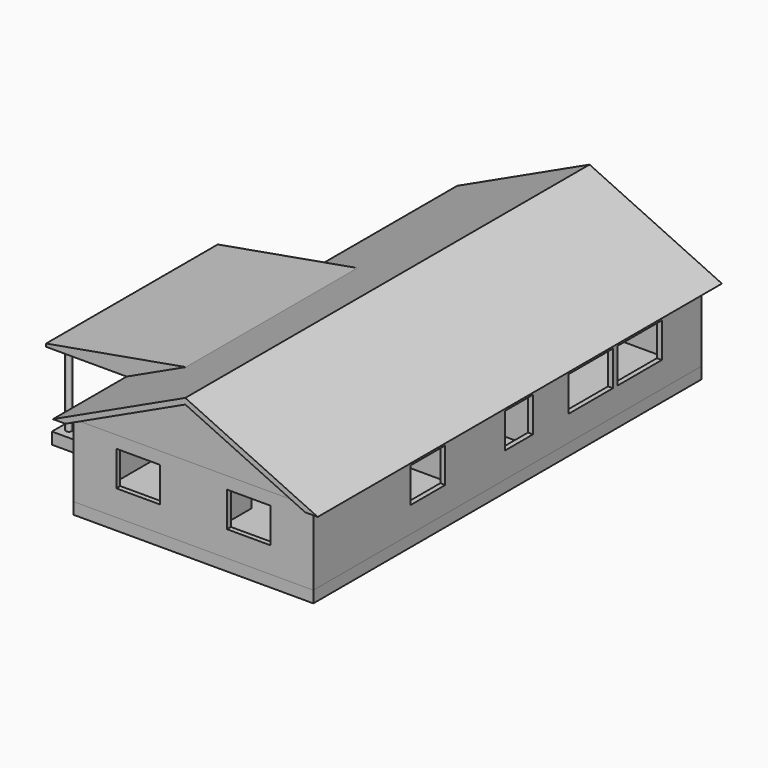
from build123d import *

# Parameters (mm, degrees)
F0_W           = 1130
F0_H           = 1950
F0_W_2         = 1120
F0_H_2         = 1100
F0_W_3         = 3760
F0_H_3         = 1500
F0_W_4         = 1710
F0_H_4         = 2010
F0_W_5         = 850
F0_H_5         = 530
F0_W_6         = 3710
F0_H_6         = 100
F1_DEPTH       = 2500
F3_START       = -400
F2_W           = 170
F2_H           = 850
F2_W_2         = 800
F2_H_2         = 150
F2_W_3         = 880
F2_H_3         = 115
F2_W_4         = 870
F2_W_5         = 850
F2_H_4         = 880
F2_W_6         = 650
F2_H_5         = 100
F2_W_7         = 160
F2_H_6         = 200
F2_W_8         = 100
F3_DEPTH       = 2100
F4_W           = 8250
F4_H           = 16680
F5_DEPTH       = 400
F6_W           = 1100
F6_H           = 650
F6_W_2         = 1350
F6_W_3         = 350
F6_H_2         = 1200
F6_W_4         = 1500
F10_DEPTH      = 170
F7_W           = 1300
F7_H           = 650
F11_DEPTH      = 200
F8_W           = 1200
F8_H           = 1200
F8_W_2         = 1900
F8_W_3         = 1500
F12_DEPTH      = 170
F9_W           = 1500
F9_H           = 1200
F13_DEPTH      = 170
F15_DEPTH      = 16680
F17_DEPTH      = 17030
F17_DEPTH_BACK = 350
F18_W          = 7380
F18_H          = 400
F19_DEPTH      = 3000
F20_W          = 1280
F20_H          = 220
F21_DEPTH      = 400
F22_R          = 100
F23_DEPTH      = 2500
F25_DEPTH      = 7380


# Not quite as in the source:
# - a feature names something its author has since deleted; it is built from what else it names


with BuildPart() as f1:
    # F0 (on Top) → F1 (new body)
    with BuildSketch(Plane.XY):
        Polygon((4125, 0), (-4125, 0), (-4125, -9510), (-3955, -9510), (-245, -9510), (-145, -9510), (3955, -9510), (4125, -9510), align=None)
        with Locations((-3390, -8335)):
            Rectangle(F0_W, F0_H, mode=Mode.SUBTRACT)
        with Locations((-2105, -6980)):
            Rectangle(F0_W_2, F0_H_2, mode=Mode.SUBTRACT)
        Polygon((-3955, -6245), (-3955, -3975), (-195, -3975), (-195, -6245), (-2825, -6245), (-2825, -7245), (-3955, -7245), align=None, mode=Mode.SUBTRACT)
        Polygon((-3955, -3860), (-3955, -1850), (-2105, -1850), (-2105, -3330), (-2105, -3860), (-2955, -3860), align=None, mode=Mode.SUBTRACT)
        with Locations((-2075, -950)):
            Rectangle(F0_W_3, F0_H_3, mode=Mode.SUBTRACT)
        with Locations((-1050, -2855)):
            Rectangle(F0_W_4, F0_H_4, mode=Mode.SUBTRACT)
        Polygon((-45, -6430), (-45, -200), (3955, -200), (3955, -5800), (1905, -5800), (1905, -6490), (3955, -6490), (3955, -9310), (955, -9310), (955, -7290), (805, -7290), (805, -9310), (-2665, -9310), (-2665, -7630), (-1415, -7630), (-1415, -6430), align=None, mode=Mode.SUBTRACT)
        with Locations((-2530, -3595)):
            Rectangle(F0_W_5, F0_H_5)
        Polygon((-145, -9510), (-245, -9510), (-245, -12960), (-245, -13060), (-245, -16510), (-145, -16510), align=None)
        with Locations((-2100, -13010)):
            Rectangle(F0_W_6, F0_H_6)
        Polygon((-3955, -9510), (-4125, -9510), (-4125, -16680), (4125, -16680), (4125, -9510), (3955, -9510), (3955, -16510), (-145, -16510), (-245, -16510), (-3955, -16510), (-3955, -13060), (-3955, -12960), align=None)
    extrude(amount=F1_DEPTH)

    # F2 (on face) → F3 (cut)
    with BuildSketch(Plane.XY.offset(2500).offset(F3_START)):
        with Locations((-4040, -1025)):
            Rectangle(F2_W, F2_H)
        with Locations((-3535, -1775)):
            Rectangle(F2_W_2, F2_H_2)
        with Locations((-3495, -3917.5)):
            Rectangle(F2_W_3, F2_H_3)
        with Locations((-640, -3917.5)):
            Rectangle(F2_W_4, F2_H_3)
        with Locations((-3330, -7302.5)):
            Rectangle(F2_W_5, F2_H_3)
        with Locations((-4040, -8420)):
            Rectangle(F2_W, F2_H_4)
        with Locations((-1890, -7580)):
            Rectangle(F2_W_6, F2_H_5)
        with Locations((-2745, -8370)):
            Rectangle(F2_W_7, F2_H_4)
        with Locations((-770, -9410)):
            Rectangle(F2_W_5, F2_H_6)
        with Locations((330, -9410)):
            Rectangle(F2_W_5, F2_H_6)
        with Locations((-195, -13585)):
            Rectangle(F2_W_8, F2_H)
    extrude(amount=-F3_DEPTH, mode=Mode.SUBTRACT)

    # F6 (on face) → F10 (cut, through all)
    with BuildSketch(Plane(origin=(-4125, 0, 0), x_dir=(0, -1, 0), z_dir=(-1, 0, 0))):
        with Locations((2760, 1775)):
            Rectangle(F6_W, F6_H)
        with Locations((5220, 1775)):
            Rectangle(F6_W_2, F6_H)
        with Locations((7565, 1450)):
            Rectangle(F6_W_3, F6_H_2)
        with Locations((11360, 1480)):
            Rectangle(F6_W_4, F6_H_2)
    extrude(amount=-F10_DEPTH, mode=Mode.SUBTRACT)

    # F7 (on face) → F11 (cut, through all)
    with BuildSketch(Plane(origin=(0, 0, 0), x_dir=(-1, 0, 0), z_dir=(0, 1, 0))):
        with Locations((1905, 1775)):
            Rectangle(F7_W, F7_H)
    extrude(amount=-F11_DEPTH, mode=Mode.SUBTRACT)

    # F8 (on face) → F12 (cut, through all)
    with BuildSketch(Plane.YZ.offset(4125)):
        with Locations((-7840, 1480)):
            Rectangle(F8_W, F8_H)
        with Locations((-4750, 1480)):
            Rectangle(F8_W_2, F8_H)
        with Locations((-2650, 1480)):
            Rectangle(F8_W_2, F8_H)
        with Locations((-11760, 1480)):
            Rectangle(F8_W_3, F8_H)
    extrude(amount=-F12_DEPTH, mode=Mode.SUBTRACT)

    # F9 (on face) → F13 (cut, through all)
    with BuildSketch(Plane.XZ.offset(16680)):
        with Locations((-1905, 1480)):
            Rectangle(F9_W, F9_H)
        with Locations((1905, 1480)):
            Rectangle(F9_W, F9_H)
    extrude(amount=-F13_DEPTH, mode=Mode.SUBTRACT)


with BuildPart() as f5:
    # F4 (on Top) → F5 (new body)
    with BuildSketch(Plane.XY):
        with Locations((0, -8340)):
            Rectangle(F4_W, F4_H)
    extrude(amount=-F5_DEPTH)


with BuildPart() as f15:
    # F14 (on face) → F15 (new body, through all)
    with BuildSketch(Plane.XZ.offset(16680)):
        Polygon((-4125, 2500), (4125, 2500), (0, 4423.5190898894), align=None)
    extrude(amount=-F15_DEPTH)


with BuildPart() as f17:
    # F16 (on face) → F17 (new body, two sides)
    with BuildSketch(Plane.XZ.offset(16680)) as f17_sk:
        Polygon((0, 4623.5190898894), (-4553.9013841019, 2500), (-4125, 2500), (0, 4423.5190898894), (4125, 2500), (4553.9013841019, 2500), align=None)
    extrude(amount=-F17_DEPTH)
    extrude(f17_sk.sketch, amount=F17_DEPTH_BACK)


with BuildPart() as f19:
    # F18 (on face) → F19 (new body)
    with BuildSketch(Plane(origin=(-4125, 0, 0), x_dir=(0, -1, 0), z_dir=(-1, 0, 0))):
        with Locations((10170, -200)):
            Rectangle(F18_W, F18_H)
    extrude(amount=F19_DEPTH)

    # F20 (on face) → F21 (join)
    with BuildSketch(Plane(origin=(-7125, 0, 0), x_dir=(0, -1, 0), z_dir=(-1, 0, 0))):
        with Locations((8420, -290)):
            Rectangle(F20_W, F20_H)
    extrude(amount=F21_DEPTH)

    # F22 (on face) → F23 (join)
    with BuildSketch(Plane.XY):
        with Locations((-6820, -6830)):
            Circle(F22_R)
        with Locations((-6820, -13510)):
            Circle(F22_R)
        with Locations((-6820, -10330)):
            Circle(F22_R)
    extrude(amount=F23_DEPTH)


with BuildPart() as f25:
    # F24 (on face) → F25 (new body, through all)
    with BuildSketch(Plane.XZ.offset(13860)):
        Polygon((-7325, 2500), (-2518.8954975725, 2500), (-2518.8954975725, 3448.9388292792), (-7325, 2600), align=None)
    extrude(amount=-F25_DEPTH)


solid = Compound([f1.part, f5.part, f15.part, f17.part, f19.part, f25.part])
